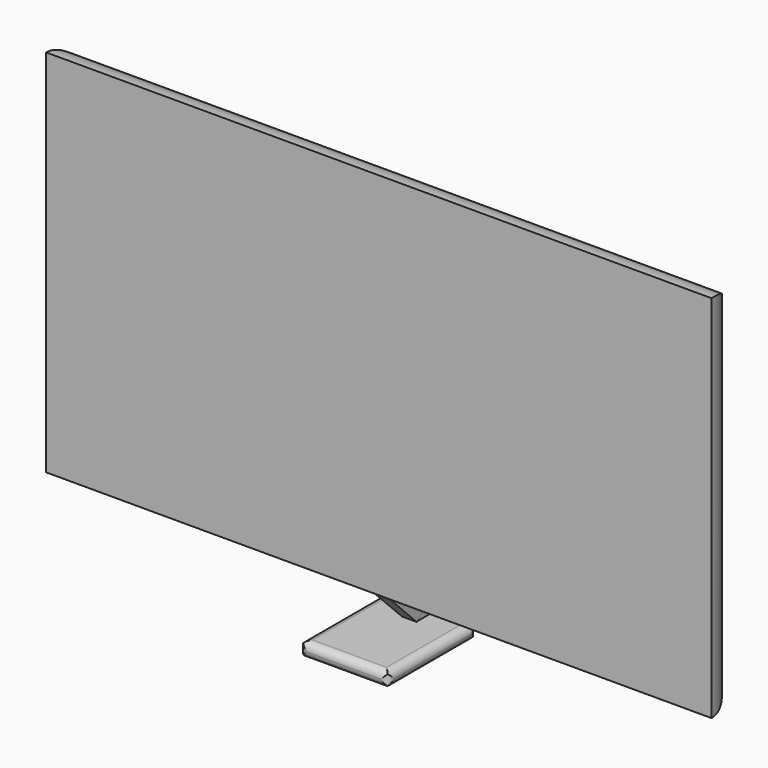
from build123d import *

# Parameters (mm, degrees)
F1_DEPTH     = 5
F3_DEPTH     = 15
F4_R         = 4.99999
F6_W         = 2
F6_H         = 5
F7_DEPTH     = 6.3
F10_DEPTH    = 9
F12_DEPTH    = 1
F13_DEPTH    = 1
F14_DEPTH    = 15
F15_R        = 0.99999
F16_T1_DEPTH = 16.00001
F16_T3_DEPTH = 7
F17_T1_DEPTH = 19
F17_T3_DEPTH = 7
F18_T1_DEPTH = 15.00001


# Not quite as in the source:
# - a fillet or chamfer that OpenCascade refuses, or shapes differently, is made with other operations: its cross-section is extruded or revolved along the edge and cut away or added
# - a fillet or chamfer is up to 0.001 mm smaller than in the source, because OpenCascade refuses the exact size


with BuildPart() as f1:
    # F0 (on Front) → F1 (new body)
    with BuildSketch(Plane.XZ):
        Polygon((45, 25), (-45, 25), (-45, -25), (-2.5, -25), (0, -25), (2.5, -25), (45, -25), align=None)
    extrude(amount=-F1_DEPTH)

    # F4 (radius 5 in the source; OpenCascade refuses exactly that, so slightly less here)
    f4_edges = [f1.edges().sort_by_distance(p)[0] for p in [
        (0, 5, 25),
        (-45, 5, 0),
        (0, 5, -25),
        (45, 5, 0),
    ]]
    fillet(f4_edges, radius=F4_R)


with BuildPart() as f3:
    # F2 (on face) → F3 (new body)
    with BuildSketch(Plane(origin=(0, 5, 0), x_dir=(-1, 0, 0), z_dir=(0, 1, 0))):
        Polygon((2.5, -30), (-2.5, -30), (-8.5, -30), (-8.5, -33), (8.5, -33), (8.5, -30), align=None)
    extrude(amount=-F3_DEPTH)


with BuildPart() as f7:
    # F6 (on face) → F7 (new body)
    with BuildSketch(Plane(origin=(0, 17.5, -17.5), x_dir=(1, 0, 0), z_dir=(0, -0.7071067812, 0.7071067812))):
        with Locations((0.0579425832, -15.0481848419)):
            Rectangle(F6_W, F6_H)
    extrude(amount=F7_DEPTH)


with BuildPart() as f10:
    # F9 (on Front) → F10 (new body)
    with BuildSketch(Plane.XZ):
        Polygon((1.0579425832, -29.9084404992), (-0.9420574168, -29.9084404992), (-5.9420574168, -29.9084404992), (-5.9420574168, -31.9084404992), (6.0579425832, -31.9084404992), (6.0579425832, -29.9084404992), align=None)
    extrude(amount=-F10_DEPTH)

    # F14 (add): a face of the model
    f14_faces = [f10.faces().sort_by_distance(p)[0] for p in [
        (0.0579425832, 9, -30.9084404992),
    ]]
    extrude(f14_faces, amount=-F14_DEPTH)

    # F15 (radius 1 in the source; OpenCascade refuses exactly that, so slightly less here)
    f15_edges = [f10.edges().sort_by_distance(p)[0] for p in [
        (6.057943, 9, -30.90844),
        (6.057943, 1.5, -29.90844),
        (6.057943, -6, -30.90844),
        (6.057943, 1.5, -31.90844),
    ]]
    fillet(f15_edges, radius=F15_R)

    # F16: fillet of radius 1 on 4 edges, made by hand

    # F16_s2 → F16_t1 (cut)
    with BuildSketch(Plane.YZ.offset(-8.4420574168)):
        with BuildLine():
            ThreePointArc((9, -30.9084404992), (8.7071067812, -30.201333718), (8, -29.9084404992))
            Line((8, -29.9084404992), (9, -29.9084404992))
            Line((9, -29.9084404992), (9, -30.9084404992))
        make_face()
        with BuildLine():
            ThreePointArc((9, -30.9084404992), (8.7071067812, -31.6155472804), (8, -31.9084404992))
            Line((8, -31.9084404992), (9, -31.9084404992))
            Line((9, -31.9084404992), (9, -30.9084404992))
        make_face()
    extrude(amount=F16_T1_DEPTH, mode=Mode.SUBTRACT)

    # F16_s4 → F16_t3 (cut)
    with BuildSketch(Plane.XY.offset(-34.4084404992)):
        with BuildLine():
            ThreePointArc((-4.9420574168, 9), (-5.649164198, 8.7071067812), (-5.9420574168, 8))
            Line((-5.9420574168, 8), (-5.9420574168, 9))
            Line((-5.9420574168, 9), (-4.9420574168, 9))
        make_face()
    extrude(amount=F16_T3_DEPTH, mode=Mode.SUBTRACT)

    # F17: fillet of radius 1 on 4 edges, made by hand

    # F17_s2 → F17_t1 (cut)
    with BuildSketch(Plane.XZ.offset(-10.5)):
        with BuildLine():
            ThreePointArc((-4.9420574168, -29.9084404992), (-5.649164198, -30.201333718), (-5.9420574168, -30.9084404992))
            Line((-5.9420574168, -30.9084404992), (-5.9420574168, -29.9084404992))
            Line((-5.9420574168, -29.9084404992), (-4.9420574168, -29.9084404992))
        make_face()
        with BuildLine():
            ThreePointArc((-4.9420574168, -31.9084404992), (-5.649164198, -31.6155472804), (-5.9420574168, -30.9084404992))
            Line((-5.9420574168, -30.9084404992), (-5.9420574168, -31.9084404992))
            Line((-5.9420574168, -31.9084404992), (-4.9420574168, -31.9084404992))
        make_face()
    extrude(amount=F17_T1_DEPTH, mode=Mode.SUBTRACT)

    # F17_s4 → F17_t3 (cut)
    with BuildSketch(Plane.XY.offset(-34.4084404992)):
        with BuildLine():
            ThreePointArc((-4.9420574168, -6), (-5.649164198, -5.7071067812), (-5.9420574168, -5))
            Line((-5.9420574168, -5), (-5.9420574168, -6))
            Line((-5.9420574168, -6), (-4.9420574168, -6))
        make_face()
    extrude(amount=F17_T3_DEPTH, mode=Mode.SUBTRACT)

    # F18: fillet of radius 1 on 4 edges, made by hand

    # F18_s2 → F18_t1 (cut)
    with BuildSketch(Plane.YZ.offset(-7.4420574168)):
        with BuildLine():
            ThreePointArc((-5, -31.9084404992), (-5.7071067812, -31.6155472804), (-6, -30.9084404992))
            Line((-6, -30.9084404992), (-6, -31.9084404992))
            Line((-6, -31.9084404992), (-5, -31.9084404992))
        make_face()
        with BuildLine():
            ThreePointArc((-5, -29.9084404992), (-5.7071067812, -30.201333718), (-6, -30.9084404992))
            Line((-6, -30.9084404992), (-6, -29.9084404992))
            Line((-6, -29.9084404992), (-5, -29.9084404992))
        make_face()
    extrude(amount=F18_T1_DEPTH, mode=Mode.SUBTRACT)


with BuildPart() as f12:
    # F11 (on Right) → F12 (new body)
    with BuildSketch(Plane.YZ):
        Polygon((8.6270934067, -29.9084404992), (8.6270934067, -26.3729065933), (5.0915595008, -29.9084404992), align=None)
    extrude(amount=F12_DEPTH)


with BuildPart() as f13:
    # F13 (new): a face of the model
    f13_faces = [f12.part.faces().sort_by_distance(p)[0] for p in [
        (0, 7.4485821048, -28.7299291972),
    ]]
    extrude(f13_faces, amount=F13_DEPTH)


solid = Compound([f1.part, f7.part, f10.part, f12.part, f13.part])
